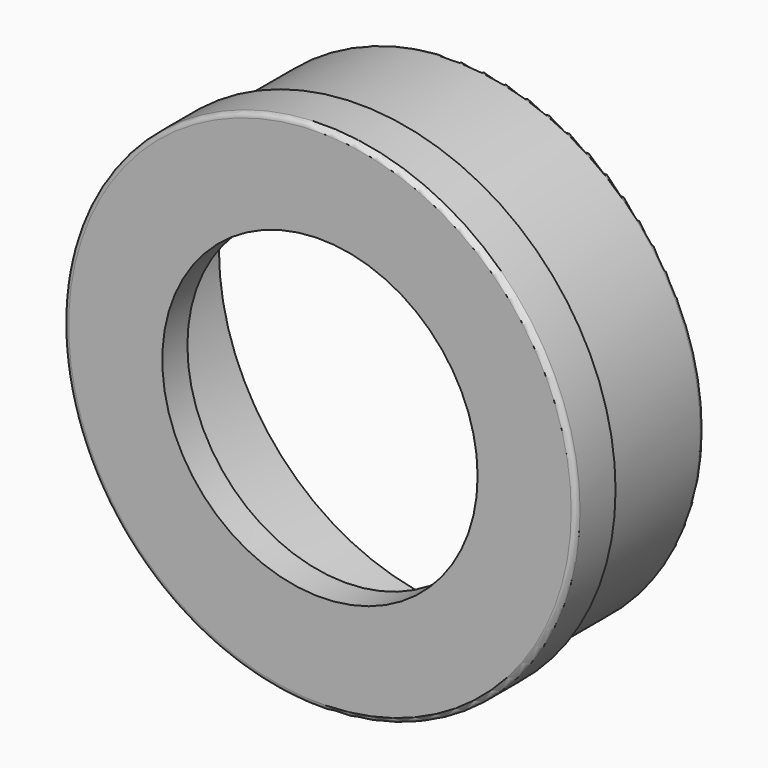
from build123d import *

# Parameters (mm, degrees)
F0_R      = 50
F1_DEPTH  = 25
F2_R      = 52
F2_R_2    = 50
F3_DEPTH  = 10
F5_T      = -1.5
F6_R      = 33.5
F6_R_2    = 31.5
F7_DEPTH  = 5
F8_R      = 1
F9_R      = 32
F10_DEPTH = 25


# Not quite as in the source:
# - a feature of the source that left no trace in its solid (it failed there, or was rolled back) is left out


with BuildPart() as f1:
    # F0 (on Front) → F1 (new body)
    with BuildSketch(Plane.XZ):
        Circle(F0_R)
    extrude(amount=F1_DEPTH)

    # F2 (on face) → F3 (join)
    with BuildSketch(Plane.XZ.offset(25)):
        Circle(F2_R)
        Circle(F2_R_2, mode=Mode.SUBTRACT)
        Circle(F2_R_2)
    extrude(amount=F3_DEPTH)

    # F5
    f5_openings = [f1.faces().sort_by_distance(p)[0] for p in [
        (0, 0, 0),
    ]]
    offset(amount=F5_T, openings=f5_openings, kind=Kind.INTERSECTION)

    # F6 (on face) → F7 (join)
    with BuildSketch(Plane(origin=(0, -33.5, 0), x_dir=(-1, 0, 0), z_dir=(0, 1, 0))):
        Circle(F6_R)
        Circle(F6_R_2, mode=Mode.SUBTRACT)
    extrude(amount=F7_DEPTH)

    # F8
    f8_edges = [f1.edges().sort_by_distance(p)[0] for p in [
        (31.5, -28.5, 0),
        (-52, -35, 0),
        (-50, 0, 0),
    ]]
    fillet(f8_edges, radius=F8_R)

    # F9 (on face) → F10 (cut)
    with BuildSketch(Plane.XZ.offset(35)):
        Circle(F9_R)
    extrude(amount=-F10_DEPTH, mode=Mode.SUBTRACT)


solid = f1.part
